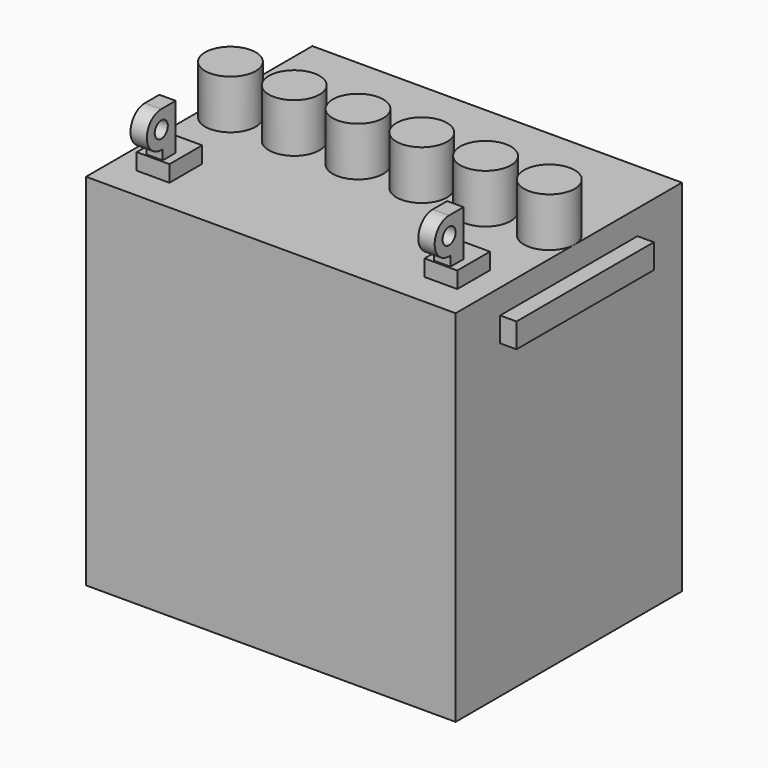
from build123d import *

# Parameters (mm, degrees)
F0_W      = 226
F0_H      = 173
F1_DEPTH  = 110
F2_W      = 105
F2_H      = 15
F3_DEPTH  = 10
F4_R      = 15.5
F5_DEPTH  = 30
F6_W      = 20
F6_H      = 25
F7_DEPTH  = 10
F10_R     = 5
F11_DEPTH = 5


# Not quite as in the source:
# - a pattern or mirror of a feature is missing from the dataset's text; its kind, count and spacing are read off the source's solid


with BuildPart() as f1:
    # F0 (on Top) → F1 (new body, symmetric)
    with BuildSketch(Plane.XY):
        Rectangle(F0_W, F0_H)
    extrude(amount=F1_DEPTH, both=True)

    # F2 (on face) → F3 (join)
    with BuildSketch(Plane(origin=(-113, 0, 0), x_dir=(0, -1, 0), z_dir=(-1, 0, 0))):
        with Locations((0, 87.5)):
            Rectangle(F2_W, F2_H)
    f3 = extrude(amount=F3_DEPTH)

    # F3_copies: F3 across plane
    add(f3.mirror(Plane(origin=(0, 0, 0), x_dir=(0, 0, 1), z_dir=(1, 0, 0))))

    # F4 (on face) → F5 (join)
    with BuildSketch(Plane.XY.offset(110)):
        with BuildLine():
            ThreePointArc((-82, 4.5), (-97.5000000043, 20), (-113, 4.4999999915))
            ThreePointArc((-113, 4.4999999915), (-97.4999999957, -11), (-82, 4.5))
        make_face()
        with Locations((-58.5, 4.5)):
            Circle(F4_R)
        with Locations((-19.5, 4.5)):
            Circle(F4_R)
        with Locations((19.5, 4.5)):
            Circle(F4_R)
        with Locations((58.5, 4.5)):
            Circle(F4_R)
        with Locations((97.5, 4.5)):
            Circle(F4_R)
    extrude(amount=F5_DEPTH)

    # F6 (on face) → F7 (join)
    with BuildSketch(Plane.XY.offset(110)):
        with Locations((88, -54)):
            Rectangle(F6_W, F6_H)
    f7 = extrude(amount=F7_DEPTH)

    # F7_copies: F7 across plane
    add(f7.mirror(Plane(origin=(0, 0, 0), x_dir=(0, 0, -1), z_dir=(-1, 0, 0))))

    # F10 (on plane+point) → F11 (join, symmetric)
    with BuildSketch(Plane.YZ.offset(88)):
        with BuildLine():
            Line((-55.4758111389, 148.0241888611), (-66.5, 148.0241888611))
            ThreePointArc((-66.5, 148.0241888611), (-77.5122627569, 136.4873509794), (-65.4758111389, 126.0234897521))
            Line((-65.4758111389, 126.0234897521), (-65.4758111389, 120))
            Line((-65.4758111389, 120), (-55.4758111389, 120))
            Line((-55.4758111389, 120), (-55.4758111389, 137))
            Line((-55.4758111389, 137), (-55.4758111389, 148.0241888611))
        make_face()
        with Locations((-66.5, 137)):
            Circle(F10_R, mode=Mode.SUBTRACT)
    f11 = extrude(amount=F11_DEPTH, both=True)

    # F11_copies: F11 across plane
    add(f11.mirror(Plane(origin=(0, 0, 0), x_dir=(0, 0, -1), z_dir=(-1, 0, 0))))


solid = f1.part
